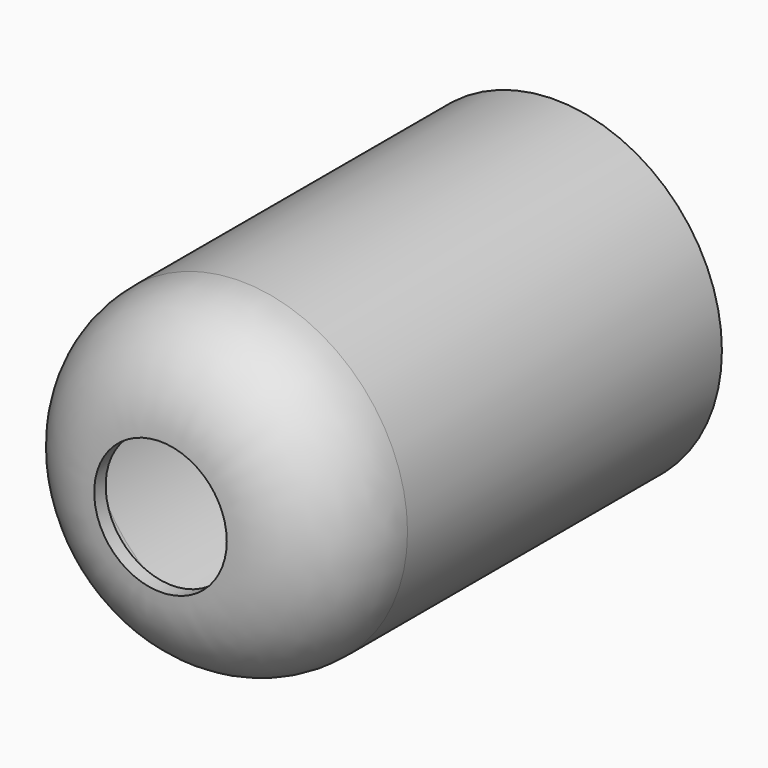
from build123d import *

# Parameters (mm, degrees)
F0_R     = 29.5216604649
F1_DEPTH = 87.376
F2_R     = 17.7830971004
F3_T     = -2.54


# Not quite as in the source:
# - a shell that OpenCascade refuses in one call is made with other operations: the cavity is built on its own and cut out


with BuildPart() as f1:
    # F0 (on Front) → F1 (new body)
    with BuildSketch(Plane.XZ):
        Circle(F0_R)
    extrude(amount=F1_DEPTH)

    # F2
    f2_edges = [f1.edges().sort_by_distance(p)[0] for p in [
        (-29.52166, -87.376, 0),
    ]]
    fillet(f2_edges, radius=F2_R)

    # F3: a shell. OpenCascade refuses it in one call, so the cavity is built on its own and cut out:
    # the body offset inwards by the wall thickness, plus a prism from it out through each open face.
    f3_core = offset(f1.part, amount=F3_T, mode=Mode.PRIVATE)
    f3_exits = [f3_core.faces().sort_by_distance(p)[0] for p in [
        (0, -84.836, 0),
    ]]
    add(f3_core, mode=Mode.SUBTRACT)
    extrude(f3_exits, amount=-F3_T, mode=Mode.SUBTRACT)


solid = f1.part
